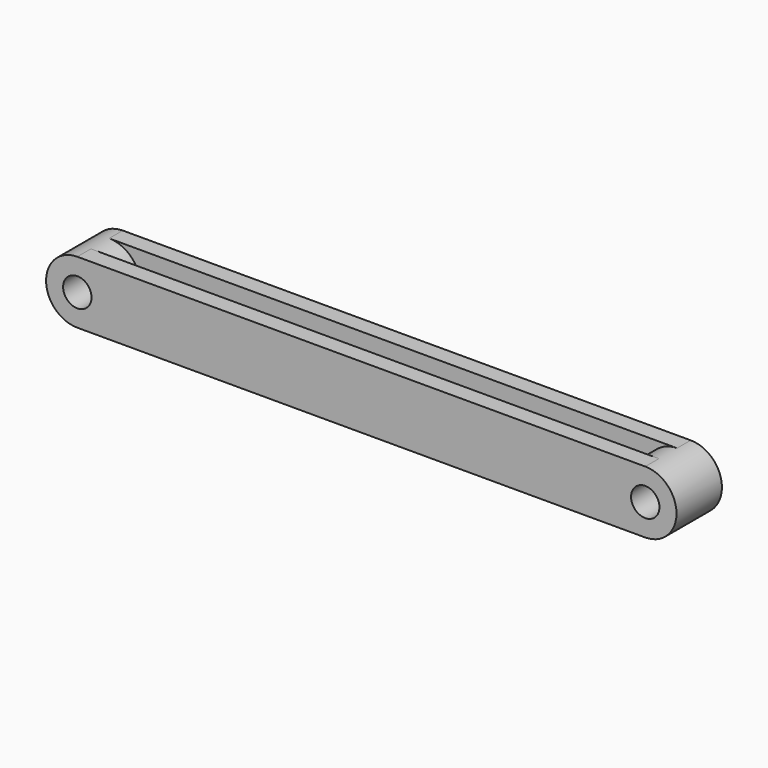
from build123d import *

# Parameters (mm, degrees)
F0_R     = 2.5
F1_DEPTH = 10
F2_T     = 3


# Not quite as in the source:
# - a shell that OpenCascade refuses in one call is made with other operations: the cavity is built on its own and cut out


with BuildPart() as f1:
    # F0 (on Front) → F1 (new body)
    with BuildSketch(Plane.XZ):
        with BuildLine():
            Line((0, 5.5), (-50, 5.5))
            ThreePointArc((-50, 5.5), (-55.5, 0), (-50, -5.5))
            Line((-50, -5.5), (0, -5.5))
            Line((0, -5.5), (50, -5.5))
            ThreePointArc((50, -5.5), (55.5, 0), (50, 5.5))
            Line((50, 5.5), (0, 5.5))
        make_face()
        with Locations((-50, 0)):
            Circle(F0_R, mode=Mode.SUBTRACT)
        with Locations((50, 0)):
            Circle(F0_R, mode=Mode.SUBTRACT)
    extrude(amount=F1_DEPTH)

    # F2: shell of thickness 3, made by hand


with BuildPart() as f2_core1:
    # F2_t2: copy of F1
    add(f1.part)

    # the walls: a layer under each face that stays
    f2_faces = [f2_core1.faces().sort_by_distance(p)[0] for p in [
        (0, -10, 0),
        (47.5, -5, 0),
        (-52.5, -5, 0),
        (55.5, -5, 0),
        (0, 0, 0),
        (-55.5, -5, 0),
    ]]
    thicken(f2_faces, amount=-F2_T, mode=Mode.SUBTRACT)


with BuildPart() as f1_1:
    add(f1.part)

    # what is left inside the walls is the cavity
    f2_cavity = [f2_core1.part.solids().sort_by_distance(p)[0] for p in [
        (0, -3.03, -1.833333),
    ]]
    add(f2_cavity, mode=Mode.SUBTRACT)


solid = f1_1.part
